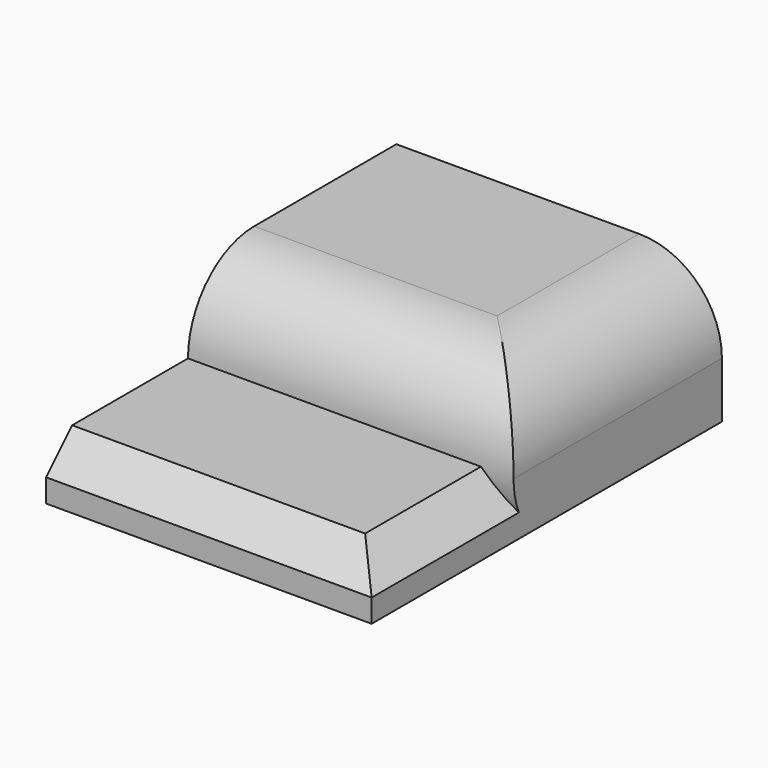
from build123d import *

# Parameters (mm, degrees)
F1_DEPTH = 8.5
F2_R     = 5.08
F3_DEPTH = 10.8966
F4_SIZE  = 2


# Not quite as in the source:
# - a feature of the source that left no trace in its solid (it failed there, or was rolled back) is left out


with BuildPart() as f1:
    # F0 (on Top) → F1 (new body)
    with BuildSketch(Plane.XY):
        with BuildLine():
            Line((8.9732294485, 7.7602798555), (-3.8267705515, 7.7602798555))
            Line((-3.8267705515, 7.7602798555), (-3.8267705515, -8.2397201445))
            ThreePointArc((-3.8267705515, -8.2397201445), (-0.2330190264, 2.0052786354), (8.9732294485, 7.7602798555))
        make_face()
        with BuildLine():
            Line((16.1732294485, 7.7602798555), (8.9732294485, 7.7602798555))
            ThreePointArc((8.9732294485, 7.7602798555), (-0.2330190264, 2.0052786354), (-3.8267705515, -8.2397201445))
            Line((-3.8267705515, -8.2397201445), (16.1732294485, -8.2397201445))
            Line((16.1732294485, -8.2397201445), (16.1732294485, 7.7602798555))
        make_face()
    extrude(amount=F1_DEPTH)

    # F2
    f2_edges = [f1.edges().sort_by_distance(p)[0] for p in [
        (16.173229, -0.23972, 8.5),
        (6.173229, -8.23972, 8.5),
    ]]
    fillet(f2_edges, radius=F2_R)

    # F3 (add): a face of the model
    f3_faces = [f1.faces().sort_by_distance(p)[0] for p in [
        (6.1732294485, -8.2397201445, 1.71),
    ]]
    extrude(f3_faces, amount=F3_DEPTH)

    # F4
    f4_edges = [f1.edges().sort_by_distance(p)[0] for p in [
        (16.173229, -13.68802, 3.42),
        (6.173229, -19.13632, 3.42),
    ]]
    chamfer(f4_edges, length=F4_SIZE)


solid = f1.part
